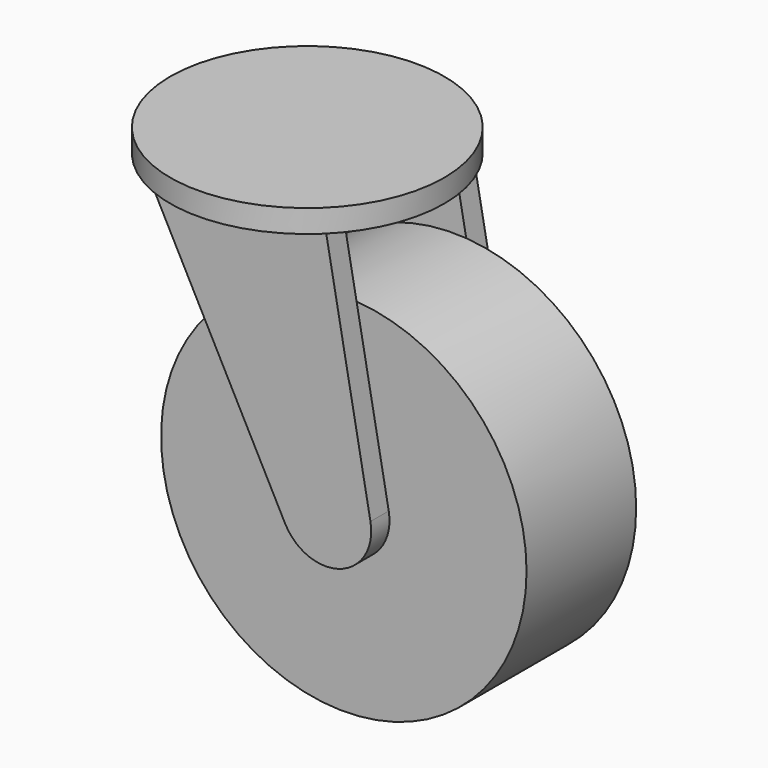
from build123d import *

# Parameters (mm, degrees)
F0_R     = 50.8
F0_R_2   = 3.175
F1_DEPTH = 19.05
F3_R     = 38.1
F4_DEPTH = 6.35
F6_DEPTH = 6.35


# Not quite as in the source:
# - a pattern or mirror of a feature is missing from the dataset's text; its kind, count and spacing are read off the source's solid


with BuildPart() as f1:
    # F0 (on Front) → F1 (new body, symmetric)
    with BuildSketch(Plane.XZ):
        Circle(F0_R)
        Circle(F0_R_2, mode=Mode.SUBTRACT)
    extrude(amount=F1_DEPTH, both=True)



with BuildPart() as f4:
    # F3 (on offset) → F4 (new body)
    with BuildSketch(Plane.XY.offset(76.2)):
        with Locations((-25.4, 0)):
            Circle(F3_R)
    extrude(amount=-F4_DEPTH)


with BuildPart() as f1_1:
    add(f1.part)

    add(f4.part)  # F6 merges F4
    # F5 (on face) → F6 (join)
    with BuildSketch(Plane(origin=(0, 19.05, 0), x_dir=(-1, 0, 0), z_dir=(0, 1, 0))):
        with BuildLine():
            Line((0, 69.85), (-12.4883185087, 2.3090909091))
            ThreePointArc((-12.4883185087, 2.3090909091), (-4.1396882106, -12.0063725379), (11.2576825912, -5.8783146118))
            Line((11.2576825912, -5.8783146118), (50.8, 69.85))
            Line((50.8, 69.85), (0, 69.85))
        make_face()
    f6 = extrude(amount=F6_DEPTH)

    # F6_copies: F6 across plane
    add(f6.mirror(Plane(origin=(0, 0, 0), x_dir=(0, 0, -1), z_dir=(0, -1, 0))))


solid = f1_1.part
